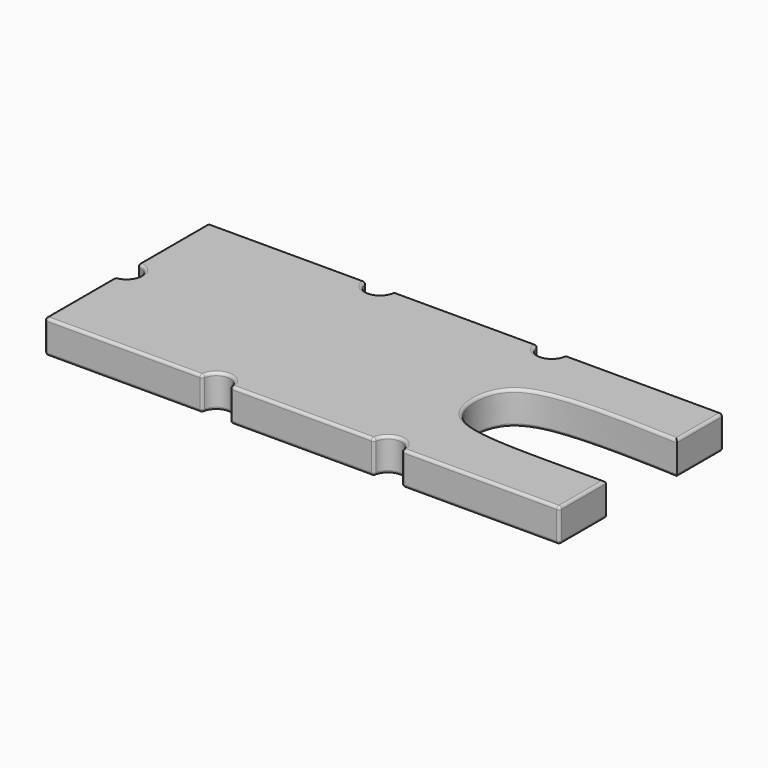
from build123d import *

# Parameters (mm, degrees)
F1_DEPTH = 3
F3_R     = 1.25
F4_R     = 1.25
F5_DEPTH = 25
F6_R     = 0.25


# Not quite as in the source:
# - a feature names something its author has since deleted; it is built from what else it names


with BuildPart() as f1:
    # F0 (on Top) → F1 (new body)
    with BuildSketch(Plane.XY):
        with BuildLine():
            Line((46.5, 0), (0, 0))
            Line((0, 0), (0, -18.5))
            Line((0, -18.5), (46.5, -18.5))
            Line((46.5, -18.5), (46.5, -13.25))
            add(Edge.make_bspline(
                [(46.5, -5.25), (41.2990462595, -5.0281633415), (34.9427373095, -4.9014690119), (31.9437700839, -6.7092677561), (31.2897903129, -9.2433737757), (31.9328215802, -11.811983406), (34.9767779409, -13.4443128539), (41.2990462595, -13.2203298325), (46.5, -13.25)],
                knots=[0, 0, 0, 0, 0.2592095959, 0.3851074736, 0.5005601093, 0.6160636246, 0.7407566781, 1, 1, 1, 1], degree=3))
            Line((46.5, -5.25), (46.5, 0))
        make_face()
    extrude(amount=F1_DEPTH)

    # F3 (on offset) + F4 (on offset) → F5 (cut)
    with BuildSketch(Plane.XY.offset(10)):
        with Locations((0, -9.25)):
            Circle(F3_R)
    with BuildSketch(Plane.XY.offset(10)):
        with Locations((15.5, 0)):
            Circle(F4_R)
        with Locations((31, 0)):
            Circle(F4_R)
        with Locations((15.5, -18.5)):
            Circle(F4_R)
        with Locations((31, -18.5)):
            Circle(F4_R)
    extrude(amount=-F5_DEPTH, mode=Mode.SUBTRACT)

    # F6
    f6_edges = [f1.edges().sort_by_distance(p)[0] for p in [
        (46.5, -2.625, 3),
        (39.375, 0, 3),
        (31, -1.25, 3),
        (23.25, 0, 3),
        (15.5, -1.25, 3),
        (7.125, 0, 3),
        (0, -4, 3),
        (1.25, -9.25, 3),
        (0, -14.5, 3),
        (7.125, -18.5, 3),
        (15.5, -17.25, 3),
        (23.25, -18.5, 3),
        (31, -17.25, 3),
        (39.375, -18.5, 3),
        (46.5, -15.875, 3),
        (31.500144, -9.220228, 3),
        (46.5, -2.625, 0),
        (39.375, 0, 0),
        (31, -1.25, 0),
        (23.25, 0, 0),
        (15.5, -1.25, 0),
        (7.125, 0, 0),
        (0, -4, 0),
        (1.25, -9.25, 0),
        (0, -14.5, 0),
        (7.125, -18.5, 0),
        (15.5, -17.25, 0),
        (23.25, -18.5, 0),
        (31, -17.25, 0),
        (39.375, -18.5, 0),
        (46.5, -15.875, 0),
        (31.500144, -9.220228, 0),
        (46.5, 0, 1.5),
        (46.5, -18.5, 1.5),
        (32.25, -18.5, 1.5),
        (29.75, -18.5, 1.5),
        (16.75, -18.5, 1.5),
        (14.25, -18.5, 1.5),
        (0, -18.5, 1.5),
        (0, -10.5, 1.5),
        (0, -8, 1.5),
        (0, 0, 1.5),
        (14.25, 0, 1.5),
        (16.75, 0, 1.5),
        (32.25, 0, 1.5),
        (29.75, 0, 1.5),
    ]]
    fillet(f6_edges, radius=F6_R)


solid = f1.part
